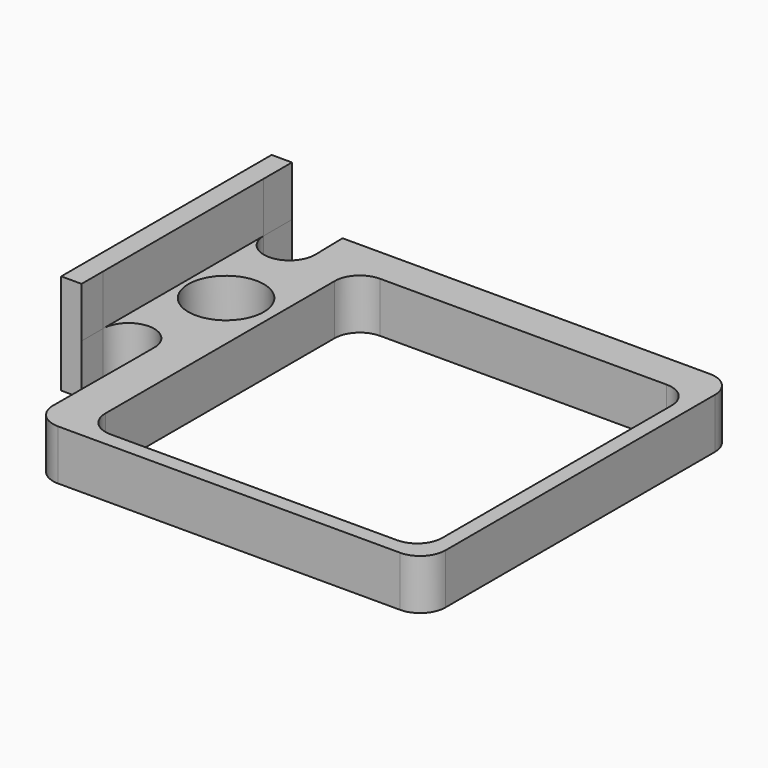
from build123d import *

# Parameters (mm, degrees)
F1_DEPTH = 10
F3_DEPTH = 10
F2_R     = 7.5
F4_DEPTH = 25


# Not quite as in the source:
# - a feature names something its author has since deleted; it is built from what else it names


with BuildPart() as f1:
    # F0 (on Top) → F1 (new body)
    with BuildSketch(Plane.XY):
        with BuildLine():
            Line((-12.3976909148, -50), (55.6003173012, -50))
            ThreePointArc((55.6003173012, -50), (59.1358512071, -48.5355339059), (60.6003173012, -45))
            Line((60.6003173012, -45), (60.6003173012, 22))
            ThreePointArc((60.6003173012, 22), (59.1358512071, 25.5355339059), (55.6003173012, 27))
            Line((55.6003173012, 27), (-17.4436509052, 27))
            Line((-17.4436509052, 27), (-17.3007774584, 20.1056662166))
            ThreePointArc((-17.3007774584, 20.1056662166), (-22.3084516237, 14.9008160564), (-27.4991044794, 19.9232047976))
            Line((-27.4991044794, 19.9232047976), (-27.4991044794, 27))
            Line((-27.4991044794, 27), (-31.5450169146, 27))
            Line((-31.5450169146, 27), (-31.5450169146, -25.2973511815))
            Line((-31.5450169146, -25.2973511815), (-27.499666141, -25.2973511815))
            Line((-27.499666141, -25.2973511815), (-27.499666141, -19.9870042568))
            ThreePointArc((-27.499666141, -19.9870042568), (-22.3611815213, -14.9001453296), (-17.3000843541, -20.0640056487))
            Line((-17.3000843541, -20.0640056487), (-17.3976909148, -45))
            ThreePointArc((-17.3976909148, -45), (-15.9332248208, -48.5355339059), (-12.3976909148, -50))
        make_face()
        with BuildLine():
            ThreePointArc((52.6003173012, 20), (56.1358512071, 18.5355339059), (57.6003173012, 15))
            Line((57.6003173012, 15), (57.6003173012, -42))
            ThreePointArc((57.6003173012, -42), (56.1358512071, -45.5355339059), (52.6003173012, -47))
            Line((52.6003173012, -47), (-4.3996826988, -47))
            ThreePointArc((-4.3996826988, -47), (-7.9352166047, -45.5355339059), (-9.3996826988, -42))
            Line((-9.3996826988, -42), (-9.3996826988, 15))
            ThreePointArc((-9.3996826988, 15), (-7.9352166047, 18.5355339059), (-4.3996826988, 20))
            Line((-4.3996826988, 20), (52.6003173012, 20))
        make_face(mode=Mode.SUBTRACT)
    extrude(amount=F1_DEPTH)

    # F2 (on face) → F3 (join)
    with BuildSketch(Plane.XY.offset(10)):
        Polygon((-27.4991044794, 27), (-31.5450169146, 27), (-31.5450169146, -25.2973511815), (-27.499666141, -25.2973511815), (-27.4996091091, -19.9870042574), (-27.4991804826, 19.9232047984), align=None)
    extrude(amount=F3_DEPTH)

    # F2 (on face) → F4 (cut)
    with BuildSketch(Plane.XY.offset(10)):
        with Locations((-19, 0)):
            Circle(F2_R)
    extrude(amount=-F4_DEPTH, mode=Mode.SUBTRACT)


solid = f1.part
